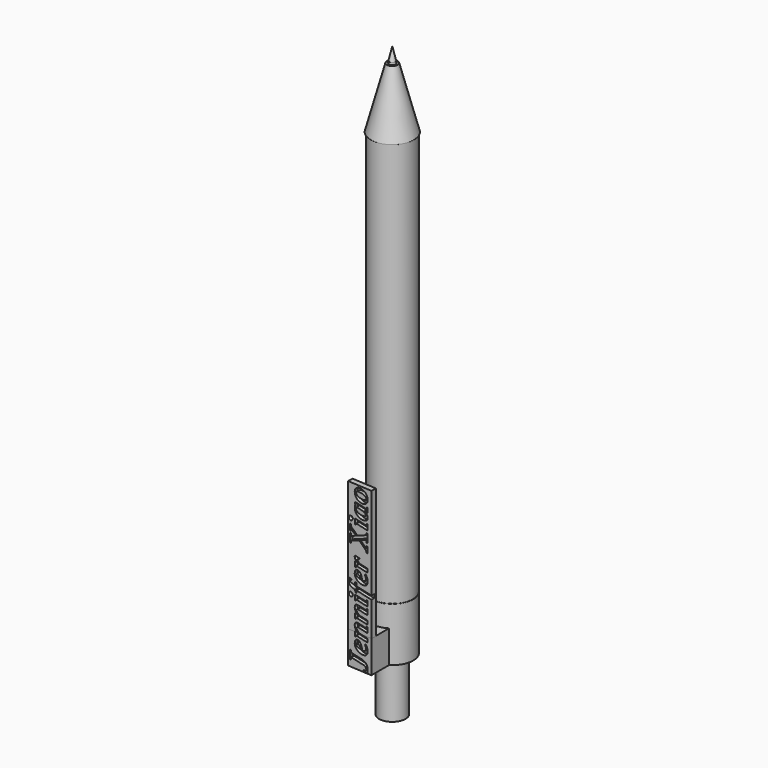
from build123d import *

# Parameters (mm, degrees)
F2_R          = 1.27
F3_DEPTH      = 25.4
F4_R          = 1.2830837913
F5_DEPTH      = 14.224
F6_R          = 0.762
F7_DEPTH      = 0.508
F10_R         = 4.8730342478
F11_DEPTH     = 95.25
F12_R         = 4.9243718978
F13_DEPTH     = 12.7
F15_DEPTH     = 7.62
F16_W         = 5.7867251092
F16_H         = 30.6203880384
F17_DEPTH     = 1.27
F18_R         = 3.112540065
F19_DEPTH     = 12.7
F20_TEXT_SIZE = 6.6793614652
F21_DEPTH     = 0.8001


# Not quite as in the source:
# - Text() gives the source's letters only with a copy of the font that has no kerning and outlines rounded to 1/6400 em; it was checked with that copy


with BuildPart() as f1:
    # F0 (on Front) → F1 (revolve)
    with BuildSketch(Plane.XZ):
        Polygon((0, 37.3435336146), (0, 56.3935336146), (-5.08, 37.3435336146), align=None)
    revolve(axis=Axis((0, 0, 46.8685336146), (0, 0, 1)))

    # F2 (on face) → F3 (cut)
    with BuildSketch(Plane(origin=(0, 0, 37.3435336146), x_dir=(1, 0, 0), z_dir=(0, 0, -1))):
        Circle(F2_R)
    extrude(amount=-F3_DEPTH, mode=Mode.SUBTRACT)

    # F4 (on face) → F5 (join)
    with BuildSketch(Plane(origin=(0, 0, 37.3435336146), x_dir=(1, 0, 0), z_dir=(0, 0, -1))):
        Circle(F4_R)
    extrude(amount=-F5_DEPTH)

    # F6 (on face) → F7 (join)
    with BuildSketch(Plane.XY.offset(51.5675336146)):
        Circle(F6_R)
    extrude(amount=F7_DEPTH)

    # F8 (on Front) → F9 (revolve)
    with BuildSketch(Plane.XZ):
        Polygon((0, 55.1308579743), (-0.7359112808, 52.0579367876), (0, 52.0579367876), align=None)
    revolve(axis=Axis((0, 0, 53.5943973809), (0, 0, -1)))

    # F10 (on face) → F11 (join)
    with BuildSketch(Plane(origin=(0, 0, 37.3435336146), x_dir=(1, 0, 0), z_dir=(0, 0, -1))):
        Circle(F10_R)
    extrude(amount=F11_DEPTH)

    # F12 (on face) → F13 (join)
    with BuildSketch(Plane(origin=(0, 0, -57.9064663854), x_dir=(1, 0, 0), z_dir=(0, 0, -1))):
        Circle(F12_R)
    extrude(amount=F13_DEPTH)

    # F14 (on face) → F15 (join)
    with BuildSketch(Plane(origin=(0, 0, -70.6064663854), x_dir=(1, 0, 0), z_dir=(0, 0, -1))):
        with BuildLine():
            Line((-3.1901652282, 9.0296297326), (-3.1901652282, 3.7513043604))
            ThreePointArc((-3.1901652282, 3.7513043604), (-0.3744624141, 4.910113694), (2.5844045003, 4.19169321))
            Line((2.5844045003, 4.19169321), (2.5844045003, 9.4045056313))
            Line((2.5844045003, 9.4045056313), (-3.1901652282, 9.0296297326))
        make_face()
    extrude(amount=-F15_DEPTH)

    # F16 (on face) → F17 (join)
    with BuildSketch(Plane(origin=(-0.5971173678, -9.1979662828, 0), x_dir=(0.997899437, -0.0647820471, 0), z_dir=(-0.0647820471, -0.997899437, 0))):
        with Locations((0.2948563682, -47.6762723662)):
            Rectangle(F16_W, F16_H)
    extrude(amount=-F17_DEPTH)

    # F18 (on face) → F19 (join)
    with BuildSketch(Plane(origin=(0, 0, -70.6064663854), x_dir=(1, 0, 0), z_dir=(0, 0, -1))):
        Circle(F18_R)
    extrude(amount=F19_DEPTH)

    # F20 (on face) → F21 (cut)
    with BuildSketch(Plane(origin=(-0.5971173678, -9.1979662828, 0), x_dir=(0.997899437, -0.0647820471, 0), z_dir=(-0.0647820471, -0.997899437, 0))):
        with Locations(Location((2.2106340685, -70.6064663854), (0, 0, 90))):
            Text('Jennifer Xiao', F20_TEXT_SIZE, font='Tinos', font_style=FontStyle.BOLDITALIC, text_align=(TextAlign.LEFT, TextAlign.BOTTOM))
    extrude(amount=-F21_DEPTH, mode=Mode.SUBTRACT)


solid = f1.part
